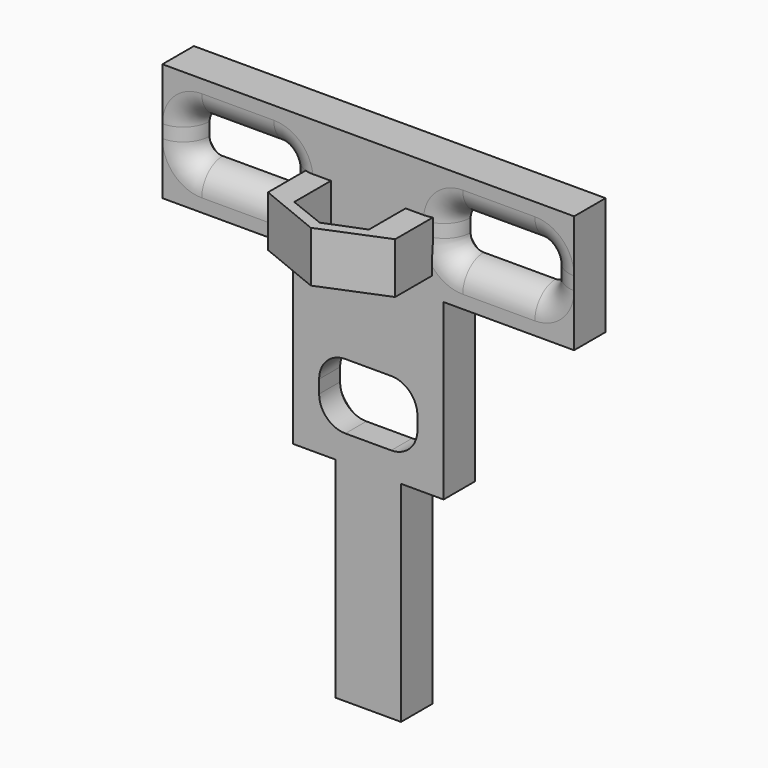
from build123d import *

# Parameters (mm, degrees)
F0_W         = 2
F0_H         = 3.8832901515
F1_DEPTH     = 3
F2_DEPTH     = 3
F2_FACE_W    = 2
F2_FACE_H    = 3.8832901515
F3_DEPTH     = 3.5
F5_DEPTH     = 3.8832901515
F6_T1_DEPTH  = 5.5
F6_T3_DEPTH  = 5.5
F6_T5_DEPTH  = 1
F6_T8_ANGLE  = 90
F6_T12_ANGLE = 90
F6_T17_DEPTH = 1
F6_T22_ANGLE = 90
F6_T28_ANGLE = 90
F6_T34_ANGLE = 90
F6_T38_ANGLE = 90
F6_T42_ANGLE = 90
F6_T45_ANGLE = 90
F6_T47_ANGLE = 90
F6_T51_ANGLE = 90
F6_T57_ANGLE = 90
F6_T63_ANGLE = 90
F6_T69_DEPTH = 1
F7_SIZE      = 0.99999


# Not quite as in the source:
# - a fillet or chamfer that OpenCascade refuses, or shapes differently, is made with other operations: its cross-section is extruded or revolved along the edge and cut away or added
# - a fillet or chamfer is up to 0.001 mm smaller than in the source, because OpenCascade refuses the exact size


with BuildPart() as f1:
    # F0 (on Front) → F1 (new body)
    with BuildSketch(Plane.XZ):
        Polygon((15.7105413526, 17.7675217465), (-5.75, 17.7675217465), (-15.7105413526, 17.7675217465), (-15.7105413526, 8.7675217465), (-5.75, 8.7675217465), (-5.75, -4.5), (-2.5, -4.5), (-2.5, -20.5), (2.5, -20.5), (2.5, -4.5), (5.75, -4.5), (5.75, 8.7675217465), (15.7105413526, 8.7675217465), (15.7105413526, 15.6582586542), align=None)
        with BuildLine():
            Line((-12.7105413526, 14.7675217465), (-7.2105413526, 14.7675217465))
            ThreePointArc((-7.2105413526, 14.7675217465), (-6.5034345714, 14.4746285276), (-6.2105413526, 13.7675217465))
            Line((-6.2105413526, 13.7675217465), (-6.2105413526, 12.7675217465))
            ThreePointArc((-6.2105413526, 12.7675217465), (-6.5034345714, 12.0604149653), (-7.2105413526, 11.7675217465))
            Line((-7.2105413526, 11.7675217465), (-12.7105413526, 11.7675217465))
            ThreePointArc((-12.7105413526, 11.7675217465), (-13.4176481338, 12.0604149653), (-13.7105413526, 12.7675217465))
            Line((-13.7105413526, 12.7675217465), (-13.7105413526, 13.7675217465))
            ThreePointArc((-13.7105413526, 13.7675217465), (-13.4176481338, 14.4746285276), (-12.7105413526, 14.7675217465))
        make_face(mode=Mode.SUBTRACT)
        with Locations((-3.85, 12.1758766707)):
            Rectangle(F0_W, F0_H, mode=Mode.SUBTRACT)
        with BuildLine():
            ThreePointArc((-3.75, 0.5), (-3.1642135624, 1.9142135624), (-1.75, 2.5))
            Line((-1.75, 2.5), (1.75, 2.5))
            ThreePointArc((1.75, 2.5), (3.1642135624, 1.9142135624), (3.75, 0.5))
            Line((3.75, 0.5), (3.75, -0.5))
            ThreePointArc((3.75, -0.5), (3.1642135624, -1.9142135624), (1.75, -2.5))
            Line((1.75, -2.5), (-1.75, -2.5))
            ThreePointArc((-1.75, -2.5), (-3.1642135624, -1.9142135624), (-3.75, -0.5))
            Line((-3.75, -0.5), (-3.75, 0.5))
        make_face(mode=Mode.SUBTRACT)
        with Locations((3.85, 12.1758766707)):
            Rectangle(F0_W, F0_H, mode=Mode.SUBTRACT)
        with BuildLine():
            ThreePointArc((7.2105413526, 11.7675217465), (6.5034345714, 12.0604149653), (6.2105413526, 12.7675217465))
            Line((6.2105413526, 12.7675217465), (6.2105413526, 13.7675217465))
            ThreePointArc((6.2105413526, 13.7675217465), (6.5034345714, 14.4746285276), (7.2105413526, 14.7675217465))
            Line((7.2105413526, 14.7675217465), (12.7105413526, 14.7675217465))
            ThreePointArc((12.7105413526, 14.7675217465), (13.4176481338, 14.4746285276), (13.7105413526, 13.7675217465))
            Line((13.7105413526, 13.7675217465), (13.7105413526, 12.7675217465))
            ThreePointArc((13.7105413526, 12.7675217465), (13.4176481338, 12.0604149653), (12.7105413526, 11.7675217465))
            Line((12.7105413526, 11.7675217465), (7.2105413526, 11.7675217465))
        make_face(mode=Mode.SUBTRACT)
    extrude(amount=F1_DEPTH)



with BuildPart() as f2:
    # F0 (on Front) → F2 (new body, through all)
    with BuildSketch(Plane.XZ):
        with Locations((-3.85, 12.1758766707)):
            Rectangle(F0_W, F0_H)
    extrude(amount=F2_DEPTH)


with BuildPart() as f2b:
    # F0 (on Front) → F2, piece 2 (new body, through all)
    with BuildSketch(Plane.XZ):
        with Locations((3.85, 12.1758766707)):
            Rectangle(F0_W, F0_H)
    extrude(amount=F2_DEPTH)


with BuildPart() as f1_1:
    add(f1.part)

    add(f2.part)  # F3 merges F2

    add(f2b.part)  # F3 merges F2b
    # F2_face (on face) → F3 (join)
    with BuildSketch(Plane(origin=(-3.85, -3, 12.1758766707), x_dir=(1, 0, 0), z_dir=(0, -1, 0))):
        Rectangle(F2_FACE_W, F2_FACE_H)
        with Locations((7.7, 0)):
            Rectangle(F2_FACE_W, F2_FACE_H)
    extrude(amount=F3_DEPTH)

    # F4 (on face) → F5 (join, through all)
    with BuildSketch(Plane(origin=(0, 0, 10.2342315949), x_dir=(1, 0, 0), z_dir=(0, 0, -1))):
        Polygon((-4.85, 6.5), (-2.85, 6.5), (0, 7.6338006184), (2.85, 6.5), (4.85, 6.5), (0, 8.4861256182), align=None)
    extrude(amount=-F5_DEPTH)

    # F6: fillet of radius 2 on 2 edges, made by hand

    # F6_s2 → F6_t1 (cut)
    with BuildSketch(Plane.YZ.offset(-12.7105413526)):
        with BuildLine():
            ThreePointArc((-1, 11.7675217465), (-2.4142135624, 11.1817353088), (-3, 9.7675217465))
            Line((-3, 9.7675217465), (-3, 11.7675217465))
            Line((-3, 11.7675217465), (-1, 11.7675217465))
        make_face()
        with BuildLine():
            ThreePointArc((-1, 14.7675217465), (-2.4142135624, 15.3533081841), (-3, 16.7675217465))
            Line((-3, 16.7675217465), (-3, 14.7675217465))
            Line((-3, 14.7675217465), (-1, 14.7675217465))
        make_face()
    extrude(amount=F6_T1_DEPTH, mode=Mode.SUBTRACT)

    # F6_s4 → F6_t3 (cut)
    with BuildSketch(Plane.YZ.offset(7.2105413526)):
        with BuildLine():
            ThreePointArc((-1, 11.7675217465), (-2.4142135624, 11.1817353088), (-3, 9.7675217465))
            Line((-3, 9.7675217465), (-3, 11.7675217465))
            Line((-3, 11.7675217465), (-1, 11.7675217465))
        make_face()
        with BuildLine():
            ThreePointArc((-1, 14.7675217465), (-2.4142135624, 15.3533081841), (-3, 16.7675217465))
            Line((-3, 16.7675217465), (-3, 14.7675217465))
            Line((-3, 14.7675217465), (-1, 14.7675217465))
        make_face()
    extrude(amount=F6_T3_DEPTH, mode=Mode.SUBTRACT)

    # F6_s6 → F6_t5 (cut)
    with BuildSketch(Plane.XY.offset(12.7675217465)):
        with BuildLine():
            ThreePointArc((13.7105413526, -1), (14.2963277903, -2.4142135624), (15.7105413526, -3))
            Line((15.7105413526, -3), (13.7105413526, -3))
            Line((13.7105413526, -3), (13.7105413526, -1))
        make_face()
        with BuildLine():
            ThreePointArc((-13.7105413526, -1), (-14.2963277903, -2.4142135624), (-15.7105413526, -3))
            Line((-15.7105413526, -3), (-13.7105413526, -3))
            Line((-13.7105413526, -3), (-13.7105413526, -1))
        make_face()
    extrude(amount=F6_T5_DEPTH, mode=Mode.SUBTRACT)

    # F6_s7 → F6_t8 (revolve, cut)
    with BuildSketch(Plane.XY.offset(12.7675217465)):
        with BuildLine():
            ThreePointArc((13.7105413526, -1), (14.2963277903, -2.4142135624), (15.7105413526, -3))
            Line((15.7105413526, -3), (13.7105413526, -3))
            Line((13.7105413526, -3), (13.7105413526, -1))
        make_face()
    revolve(axis=Axis((12.7105413526, -3, 12.7675217465), (0, 1, 0)), revolution_arc=F6_T8_ANGLE, mode=Mode.SUBTRACT)


with BuildPart() as f6_tool10:
    # F6_s11 → F6_t12 (revolve)
    with BuildSketch(Plane.YZ.offset(7.2105413526)):
        with BuildLine():
            ThreePointArc((-1, 11.7675217465), (-2.4142135624, 11.1817353088), (-3, 9.7675217465))
            Line((-3, 9.7675217465), (-3, 11.7675217465))
            Line((-3, 11.7675217465), (-1, 11.7675217465))
        make_face()
    revolve(axis=Axis((7.2105413526, -3, 12.7675217465), (0, 1, 0)), revolution_arc=F6_T12_ANGLE)

    split(bisect_by=Plane.YZ.offset(4.85), keep=Keep.TOP)


with BuildPart() as f1_2:
    add(f1_1.part)

    # F6_t9: cut F6_tool10
    add(f6_tool10.part, mode=Mode.SUBTRACT)


with BuildPart() as f6_tool15:
    # F6_s16 → F6_t17 (new body)
    with BuildSketch(Plane.XY.offset(12.7675217465)):
        with BuildLine():
            ThreePointArc((6.2105413526, -1), (5.624754915, -2.4142135624), (4.2105413526, -3))
            Line((4.2105413526, -3), (6.2105413526, -3))
            Line((6.2105413526, -3), (6.2105413526, -1))
        make_face()
    extrude(amount=F6_T17_DEPTH)

    split(bisect_by=Plane.YZ.offset(4.85), keep=Keep.TOP)


with BuildPart() as f1_3:
    add(f1_2.part)

    # F6_t14: cut F6_tool15
    add(f6_tool15.part, mode=Mode.SUBTRACT)


with BuildPart() as f6_tool20:
    # F6_s21 → F6_t22 (revolve)
    with BuildSketch(Plane.XY.offset(13.7675217465)):
        with BuildLine():
            ThreePointArc((6.2105413526, -1), (5.624754915, -2.4142135624), (4.2105413526, -3))
            Line((4.2105413526, -3), (6.2105413526, -3))
            Line((6.2105413526, -3), (6.2105413526, -1))
        make_face()
    revolve(axis=Axis((7.2105413526, -3, 13.7675217465), (0, 1, 0)), revolution_arc=F6_T22_ANGLE)

    split(bisect_by=Plane.XY.offset(14.1175217465), keep=Keep.BOTTOM)

    split(bisect_by=Plane.YZ.offset(4.85), keep=Keep.TOP)


with BuildPart() as f1_4:
    add(f1_3.part)

    # F6_t19: cut F6_tool20
    add(f6_tool20.part, mode=Mode.SUBTRACT)


with BuildPart() as f6_tool26:
    # F6_s27 → F6_t28 (revolve)
    with BuildSketch(Plane.XY.offset(13.7675217465)):
        with BuildLine():
            ThreePointArc((6.2105413526, -1), (5.624754915, -2.4142135624), (4.2105413526, -3))
            Line((4.2105413526, -3), (6.2105413526, -3))
            Line((6.2105413526, -3), (6.2105413526, -1))
        make_face()
    revolve(axis=Axis((7.2105413526, -3, 13.7675217465), (0, 1, 0)), revolution_arc=F6_T28_ANGLE)

    split(bisect_by=Plane.XY.offset(14.1175217465), keep=Keep.TOP)

    split(bisect_by=Plane.YZ.offset(4.85), keep=Keep.TOP)


with BuildPart() as f1_5:
    add(f1_4.part)

    # F6_t25: cut F6_tool26
    add(f6_tool26.part, mode=Mode.SUBTRACT)


with BuildPart() as f6_tool32:
    # F6_s33 → F6_t34 (revolve)
    with BuildSketch(Plane.XY.offset(13.7675217465)):
        with BuildLine():
            ThreePointArc((6.2105413526, -1), (5.624754915, -2.4142135624), (4.2105413526, -3))
            Line((4.2105413526, -3), (6.2105413526, -3))
            Line((6.2105413526, -3), (6.2105413526, -1))
        make_face()
    revolve(axis=Axis((7.2105413526, -3, 13.7675217465), (0, 1, 0)), revolution_arc=F6_T34_ANGLE)

    split(bisect_by=Plane.XY.offset(14.1175217465), keep=Keep.TOP)

    split(bisect_by=Plane.YZ.offset(4.85), keep=Keep.BOTTOM)


with BuildPart() as f1_6:
    add(f1_5.part)

    # F6_t31: cut F6_tool32
    add(f6_tool32.part, mode=Mode.SUBTRACT)

    # F6_s37 → F6_t38 (revolve, cut)
    with BuildSketch(Plane.YZ.offset(12.7105413526)):
        with BuildLine():
            ThreePointArc((-1, 14.7675217465), (-2.4142135624, 15.3533081841), (-3, 16.7675217465))
            Line((-3, 16.7675217465), (-3, 14.7675217465))
            Line((-3, 14.7675217465), (-1, 14.7675217465))
        make_face()
    revolve(axis=Axis((12.7105413526, -3, 13.7675217465), (0, 1, 0)), revolution_arc=F6_T38_ANGLE, mode=Mode.SUBTRACT)


with BuildPart() as f6_tool40:
    # F6_s41 → F6_t42 (revolve)
    with BuildSketch(Plane.XY.offset(12.7675217465)):
        with BuildLine():
            ThreePointArc((-6.2105413526, -1), (-5.624754915, -2.4142135624), (-4.2105413526, -3))
            Line((-4.2105413526, -3), (-6.2105413526, -3))
            Line((-6.2105413526, -3), (-6.2105413526, -1))
        make_face()
    revolve(axis=Axis((-7.2105413526, -3, 12.7675217465), (0, 1, 0)), revolution_arc=F6_T42_ANGLE)

    split(bisect_by=Plane.YZ.offset(-4.85), keep=Keep.BOTTOM)


with BuildPart() as f1_7:
    add(f1_6.part)

    # F6_t39: cut F6_tool40
    add(f6_tool40.part, mode=Mode.SUBTRACT)

    # F6_s44 → F6_t45 (revolve, cut)
    with BuildSketch(Plane.YZ.offset(-12.7105413526)):
        with BuildLine():
            ThreePointArc((-1, 11.7675217465), (-2.4142135624, 11.1817353088), (-3, 9.7675217465))
            Line((-3, 9.7675217465), (-3, 11.7675217465))
            Line((-3, 11.7675217465), (-1, 11.7675217465))
        make_face()
    revolve(axis=Axis((-12.7105413526, -3, 12.7675217465), (0, 1, 0)), revolution_arc=F6_T45_ANGLE, mode=Mode.SUBTRACT)

    # F6_s46 → F6_t47 (revolve, cut)
    with BuildSketch(Plane.XY.offset(13.7675217465)):
        with BuildLine():
            ThreePointArc((-13.7105413526, -1), (-14.2963277903, -2.4142135624), (-15.7105413526, -3))
            Line((-15.7105413526, -3), (-13.7105413526, -3))
            Line((-13.7105413526, -3), (-13.7105413526, -1))
        make_face()
    revolve(axis=Axis((-12.7105413526, -3, 13.7675217465), (0, 1, 0)), revolution_arc=F6_T47_ANGLE, mode=Mode.SUBTRACT)


with BuildPart() as f6_tool49:
    # F6_s50 → F6_t51 (revolve)
    with BuildSketch(Plane.YZ.offset(-7.2105413526)):
        with BuildLine():
            ThreePointArc((-1, 14.7675217465), (-2.4142135624, 15.3533081841), (-3, 16.7675217465))
            Line((-3, 16.7675217465), (-3, 14.7675217465))
            Line((-3, 14.7675217465), (-1, 14.7675217465))
        make_face()
    revolve(axis=Axis((-7.2105413526, -3, 13.7675217465), (0, 1, 0)), revolution_arc=F6_T51_ANGLE)

    split(bisect_by=Plane.XY.offset(14.1175217465), keep=Keep.TOP)

    split(bisect_by=Plane.YZ.offset(-4.85), keep=Keep.BOTTOM)


with BuildPart() as f1_8:
    add(f1_7.part)

    # F6_t48: cut F6_tool49
    add(f6_tool49.part, mode=Mode.SUBTRACT)


with BuildPart() as f6_tool55:
    # F6_s56 → F6_t57 (revolve)
    with BuildSketch(Plane.YZ.offset(-7.2105413526)):
        with BuildLine():
            ThreePointArc((-1, 14.7675217465), (-2.4142135624, 15.3533081841), (-3, 16.7675217465))
            Line((-3, 16.7675217465), (-3, 14.7675217465))
            Line((-3, 14.7675217465), (-1, 14.7675217465))
        make_face()
    revolve(axis=Axis((-7.2105413526, -3, 13.7675217465), (0, 1, 0)), revolution_arc=F6_T57_ANGLE)

    split(bisect_by=Plane.XY.offset(14.1175217465), keep=Keep.TOP)

    split(bisect_by=Plane.YZ.offset(-4.85), keep=Keep.TOP)


with BuildPart() as f1_9:
    add(f1_8.part)

    # F6_t54: cut F6_tool55
    add(f6_tool55.part, mode=Mode.SUBTRACT)


with BuildPart() as f6_tool61:
    # F6_s62 → F6_t63 (revolve)
    with BuildSketch(Plane.YZ.offset(-7.2105413526)):
        with BuildLine():
            ThreePointArc((-1, 14.7675217465), (-2.4142135624, 15.3533081841), (-3, 16.7675217465))
            Line((-3, 16.7675217465), (-3, 14.7675217465))
            Line((-3, 14.7675217465), (-1, 14.7675217465))
        make_face()
    revolve(axis=Axis((-7.2105413526, -3, 13.7675217465), (0, 1, 0)), revolution_arc=F6_T63_ANGLE)

    split(bisect_by=Plane.XY.offset(14.1175217465), keep=Keep.BOTTOM)

    split(bisect_by=Plane.YZ.offset(-4.85), keep=Keep.BOTTOM)


with BuildPart() as f1_10:
    add(f1_9.part)

    # F6_t60: cut F6_tool61
    add(f6_tool61.part, mode=Mode.SUBTRACT)


with BuildPart() as f6_tool67:
    # F6_s68 → F6_t69 (new body)
    with BuildSketch(Plane.XY.offset(13.7675217465)):
        with BuildLine():
            ThreePointArc((-6.2105413526, -1), (-5.624754915, -2.4142135624), (-4.2105413526, -3))
            Line((-4.2105413526, -3), (-6.2105413526, -3))
            Line((-6.2105413526, -3), (-6.2105413526, -1))
        make_face()
    extrude(amount=-F6_T69_DEPTH)

    split(bisect_by=Plane.YZ.offset(-4.85), keep=Keep.BOTTOM)


with BuildPart() as f1_11:
    add(f1_10.part)

    # F6_t66: cut F6_tool67
    add(f6_tool67.part, mode=Mode.SUBTRACT)

    # F7 (size 1 in the source; OpenCascade refuses exactly that, so slightly less here)
    f7_edges = [f1_11.edges().sort_by_distance(p)[0] for p in [
        (-9.960541, 0, 11.767522),
        (6.503435, 0, 14.474629),
        (0, 0, 2.5),
    ]]
    chamfer(f7_edges, length=F7_SIZE)


solid = f1_11.part
